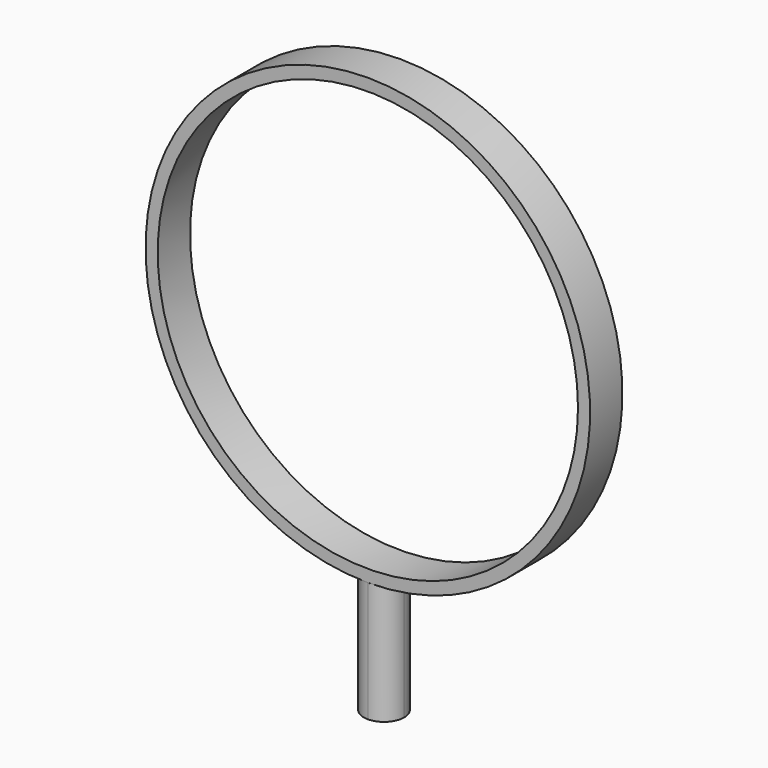
from build123d import *

# Parameters (mm, degrees)
F0_R     = 52
F1_DEPTH = 10
F2_R     = 4.99999


# Not quite as in the source:
# - a fillet or chamfer is up to 0.001 mm smaller than in the source, because OpenCascade refuses the exact size


with BuildPart() as f1:
    # F0 (on Front) → F1 (new body)
    with BuildSketch(Plane.XZ):
        with BuildLine():
            Line((5, -84.7722557505), (5, -54.7722557505))
            ThreePointArc((5, -54.7722557505), (0, 55), (-5, -54.7722557505))
            Line((-5, -54.7722557505), (-5, -84.7722557505))
            Line((-5, -84.7722557505), (5, -84.7722557505))
        make_face()
        Circle(F0_R, mode=Mode.SUBTRACT)
    extrude(amount=F1_DEPTH)

    # F2 (radius 5 in the source; OpenCascade refuses exactly that, so slightly less here)
    f2_edges = [f1.edges().sort_by_distance(p)[0] for p in [
        (5, -10, -69.772256),
        (-5, -10, -69.772256),
        (-5, 0, -69.772256),
        (5, 0, -69.772256),
    ]]
    fillet(f2_edges, radius=F2_R)


solid = f1.part
